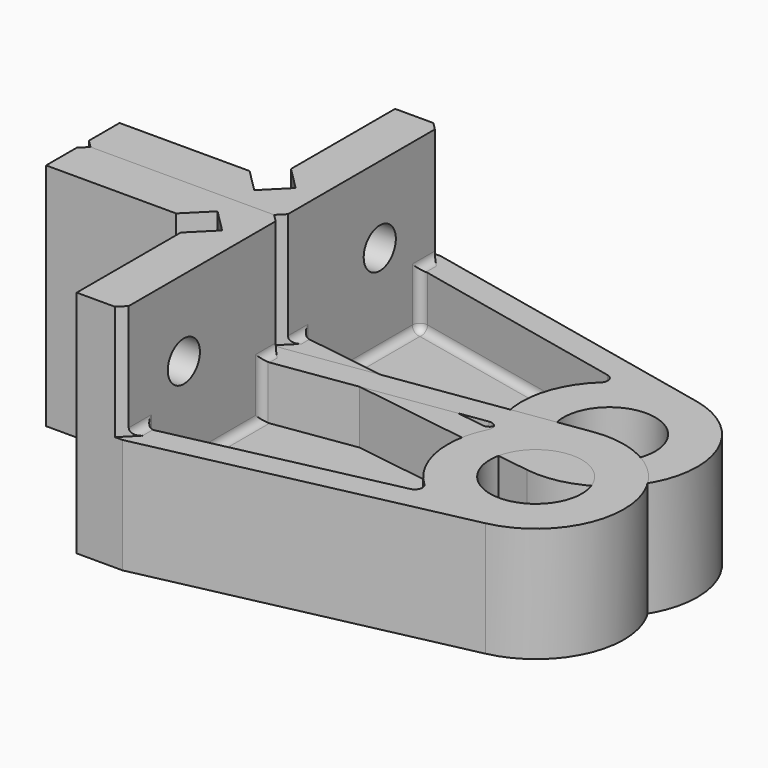
from build123d import *

# Parameters (mm, degrees)
F1_R      = 6
F2_DEPTH  = 8
F3_R      = 6
F4_DEPTH  = 15
F6_DEPTH  = 30
F7_SIZE   = 1
F8_R      = 1
F9_R      = 8.125
F10_DEPTH = 5
F11_R     = 2.625
F12_DEPTH = 11.501
F13_R     = 2.625
F14_DEPTH = 6


with BuildPart() as f2:
    # F1 (on Top) → F2 (new body)
    with BuildSketch(Plane.XY):
        with BuildLine():
            ThreePointArc((-1.6840484339, -11.3760265854), (11.3138603774, -2.0607191369), (2.4351188346, 11.2392257857))
            Line((2.4351188346, 11.2392257857), (-38, 20))
            Line((-38, 20), (-38, -6))
            Line((-38, -6), (-1.6840484339, -11.3760265854))
        make_face()
        Circle(F1_R, mode=Mode.SUBTRACT)
    extrude(amount=F2_DEPTH)

    # F3 (on Top) → F4 (join)
    with BuildSketch(Plane.XY):
        with BuildLine():
            Line((-38, 16.5466927402), (-6.2334383583, 9.6640698587))
            ThreePointArc((-6.2334383583, 9.6640698587), (-11.3138603774, 2.0607191369), (-9.2405323218, -6.8456235954))
            Line((-9.2405323218, -6.8456235954), (-38, -2.5882199986))
            Line((-38, -2.5882199986), (-38, -6))
            Line((-38, -6), (-1.6840484339, -11.3760265854))
            ThreePointArc((-1.6840484339, -11.3760265854), (11.3138603774, -2.0607191369), (2.4351188346, 11.2392257857))
            Line((2.4351188346, 11.2392257857), (-38, 20))
            Line((-38, 20), (-38, 16.5466927402))
        make_face()
        Circle(F3_R, mode=Mode.SUBTRACT)
    extrude(amount=F4_DEPTH)

    # F5 (on Top) → F6 (join)
    with BuildSketch(Plane.XY):
        Polygon((-38, -6), (-38, 20), (-44, 20), (-44, 3.00520382), (-40.99479618, 0), (-44, -3.00520382), (-47.00520382, 0), (-64, 0), (-64, -6), align=None)
    extrude(amount=F6_DEPTH)

    # F7
    f7_edges = [f2.edges().sort_by_distance(p)[0] for p in [
        (-64, -6, 15),
        (-38, 20, 22.5),
        (-38, -6, 22.5),
    ]]
    chamfer(f7_edges, length=F7_SIZE)

    # F8
    f8_edges = [f2.edges().sort_by_distance(p)[0] for p in [
        (-22.116719, 13.105381, 8),
        (-38, 6.979236, 8),
        (-38, -3.79411, 15),
        (-38, 17.773346, 15),
        (-11.31386, 2.060719, 8),
        (-6.233438, 9.66407, 11.5),
        (-9.240532, -6.845624, 11.5),
        (-38, 16.546693, 11.5),
        (-38, -2.58822, 11.5),
    ]]
    fillet(f8_edges, radius=F8_R)

    # F9 (on face) → F10 (cut)
    with BuildSketch(Plane(origin=(0, 0, 0), x_dir=(1, 0, 0), z_dir=(0, 0, -1))):
        Circle(F9_R)
    extrude(amount=-F10_DEPTH, mode=Mode.SUBTRACT)

    # F11 (on face) → F12 (cut, through all)
    with BuildSketch(Plane(origin=(0, 0, 0), x_dir=(-1, 0, 0), z_dir=(0, 1, 0))):
        with Locations((54, 10)):
            Circle(F11_R)
    extrude(amount=-F12_DEPTH, mode=Mode.SUBTRACT)

    # F13 (on face) → F14 (cut, through all)
    with BuildSketch(Plane(origin=(-44, 0, 0), x_dir=(0, -1, 0), z_dir=(-1, 0, 0))):
        with Locations((-10, 20)):
            Circle(F13_R)
    extrude(amount=-F14_DEPTH, mode=Mode.SUBTRACT)


with BuildPart() as f15_1:
    # F15: instance of F2
    add(f2.part.mirror(Plane(origin=(-50.64611798, -6, 14.9940249514), x_dir=(1, 0, 0), z_dir=(0, -1, 0))))


solid = Compound([f2.part, f15_1.part])
